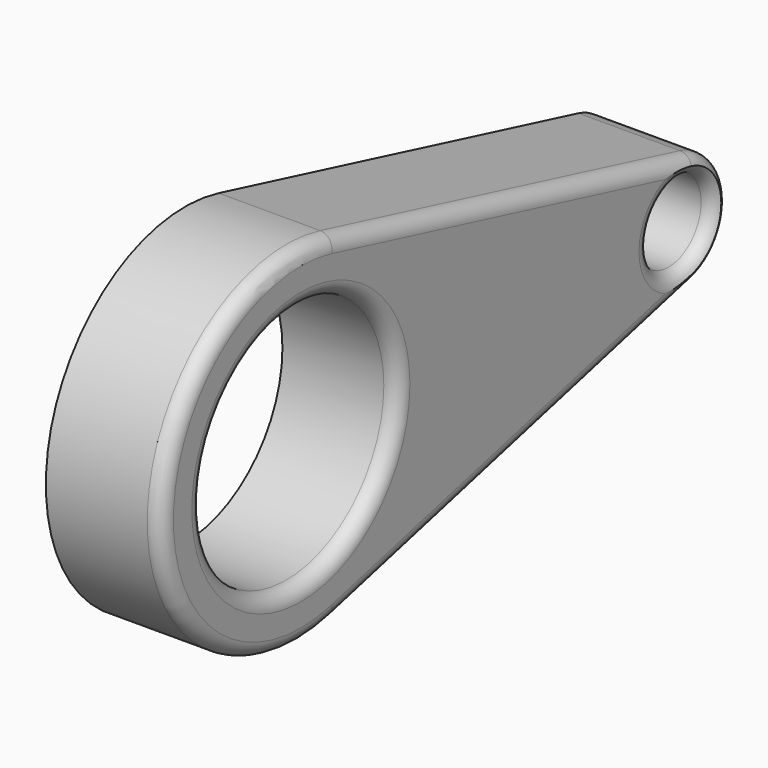
from build123d import *

# Parameters (mm, degrees)
F1_DEPTH    = 20
F2_R        = 7.0042863138
F2_R_2      = 21.0298639767
F3_DEPTH    = 20
F4_T1_DEPTH = 80
F4_T3_DEPTH = 80
F4_T6_ANGLE = 208.0724869359
F4_T8_ANGLE = 151.9275130641
F5_T        = -0.5


# Not quite as in the source:
# - a fillet or chamfer that OpenCascade refuses, or shapes differently, is made with other operations: its cross-section is extruded or revolved along the edge and cut away or added


with BuildPart() as f1:
    # F0 (on Right) → F1 (new body)
    with BuildSketch(Plane.YZ):
        with BuildLine():
            ThreePointArc((7.2760687511, -29.1042750044), (23.6461631405, -18.4623662821), (30, 0))
            ThreePointArc((30, 0), (23.6461631405, 18.4623662821), (7.2760687511, 29.1042750044))
            ThreePointArc((7.2760687511, 29.1042750044), (-30, 0), (7.2760687511, -29.1042750044))
        make_face()
        with BuildLine():
            ThreePointArc((7.2760687511, 29.1042750044), (23.6461631405, 18.4623662821), (30, 0))
            ThreePointArc((30, 0), (23.6461631405, -18.4623662821), (7.2760687511, -29.1042750044))
            Line((7.2760687511, -29.1042750044), (84.8874687627, -9.7014250015))
            ThreePointArc((84.8874687627, -9.7014250015), (72.4621125124, 0), (84.8874687627, 9.7014250015))
            Line((84.8874687627, 9.7014250015), (7.2760687511, 29.1042750044))
        make_face()
        with BuildLine():
            ThreePointArc((92.4621125124, 0), (90.3441668925, 6.154122094), (84.8874687627, 9.7014250015))
            ThreePointArc((84.8874687627, 9.7014250015), (72.4621125124, 0), (84.8874687627, -9.7014250015))
            ThreePointArc((84.8874687627, -9.7014250015), (90.3441668925, -6.154122094), (92.4621125124, 0))
        make_face()
    extrude(amount=F1_DEPTH)

    # F2 (on face) → F3 (cut)
    with BuildSketch(Plane.YZ.offset(20)):
        with Locations((82.4621125124, 0)):
            Circle(F2_R)
        Circle(F2_R_2)
    extrude(amount=-F3_DEPTH, mode=Mode.SUBTRACT)

    # F4: fillet of radius 2.5 on 6 edges, made by hand

    # F4_s2 → F4_t1 (cut)
    with BuildSketch(Plane(origin=(0, 77.6114000116, -19.4028500029), x_dir=(1, 0, 0), z_dir=(0, -0.9701425001, 0.242535625))):
        with BuildLine():
            ThreePointArc((17.5, 30), (19.267766953, 29.267766953), (20, 27.5))
            Line((20, 27.5), (20, 30))
            Line((20, 30), (17.5, 30))
        make_face()
    extrude(amount=F4_T1_DEPTH, mode=Mode.SUBTRACT)

    # F4_s4 → F4_t3 (cut)
    with BuildSketch(Plane(origin=(0, 0, 0), x_dir=(1, 0, 0), z_dir=(0, 0.9701425001, 0.242535625))):
        with BuildLine():
            ThreePointArc((17.5, 30), (19.267766953, 29.267766953), (20, 27.5))
            Line((20, 27.5), (20, 30))
            Line((20, 30), (17.5, 30))
        make_face()
    extrude(amount=F4_T3_DEPTH, mode=Mode.SUBTRACT)

    # F4_s5 → F4_t6 (revolve, cut)
    with BuildSketch(Plane(origin=(0, 0, 0), x_dir=(1, 0, 0), z_dir=(0, 0.9701425001, -0.242535625))):
        with BuildLine():
            ThreePointArc((17.5, -30), (19.267766953, -29.267766953), (20, -27.5))
            Line((20, -27.5), (20, -30))
            Line((20, -30), (17.5, -30))
        make_face()
    revolve(axis=Axis((20, 0, 0), (1, 0, 0)), revolution_arc=F4_T6_ANGLE, mode=Mode.SUBTRACT)

    # F4_s7 → F4_t8 (revolve, cut)
    with BuildSketch(Plane(origin=(0, 77.6114000116, 19.4028500029), x_dir=(1, 0, 0), z_dir=(0, -0.9701425001, -0.242535625))):
        with BuildLine():
            ThreePointArc((20, -27.5), (19.267766953, -29.267766953), (17.5, -30))
            Line((17.5, -30), (20, -30))
            Line((20, -30), (20, -27.5))
        make_face()
    revolve(axis=Axis((20, 82.4621125124, 0), (1, 0, 0)), revolution_arc=F4_T8_ANGLE, mode=Mode.SUBTRACT)

    # F4_s9 → F4_t10 (revolve, cut)
    with BuildSketch(Plane.XY):
        with BuildLine():
            ThreePointArc((20, 23.5298639767), (19.267766953, 21.7620970238), (17.5, 21.0298639767))
            Line((17.5, 21.0298639767), (20, 21.0298639767))
            Line((20, 21.0298639767), (20, 23.5298639767))
        make_face()
    revolve(axis=Axis((20, 0, 0), (1, 0, 0)), mode=Mode.SUBTRACT)

    # F4_s11 → F4_t12 (revolve, cut)
    with BuildSketch(Plane.XY):
        with BuildLine():
            ThreePointArc((20, 91.9663988262), (19.267766953, 90.1986318732), (17.5, 89.4663988262))
            Line((17.5, 89.4663988262), (20, 89.4663988262))
            Line((20, 89.4663988262), (20, 91.9663988262))
        make_face()
    revolve(axis=Axis((20, 82.4621125124, 0), (1, 0, 0)), mode=Mode.SUBTRACT)

    # F5
    f5_openings = [f1.faces().sort_by_distance(p)[0] for p in [
        (0, 29.143198, 0),
    ]]
    offset(amount=F5_T, openings=f5_openings)


solid = f1.part
